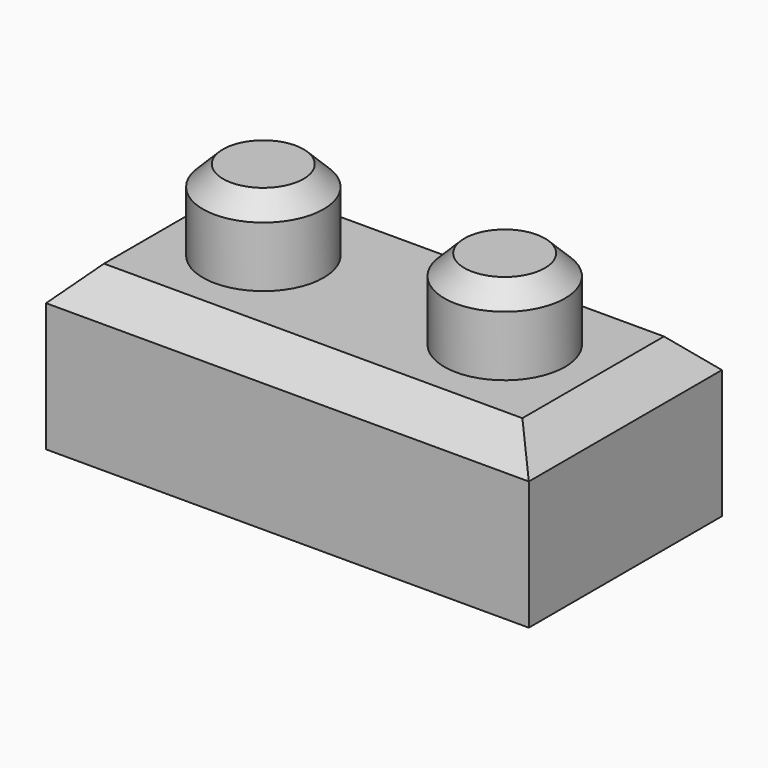
from build123d import *

# Parameters (mm, degrees)
F0_W     = 76.2
F0_H     = 38.1
F1_DEPTH = 25.4
F2_SIZE  = 5.08
F3_R     = 9.525
F4_DEPTH = 12.7
F5_SIZE2 = 3.175
F5_SIZE  = 3.175
F6_T     = 7.9375


# Not quite as in the source:
# - a shell that OpenCascade refuses in one call is made with other operations: the cavity is built on its own and cut out


with BuildPart() as f1:
    # F0 (on Top) → F1 (new body)
    with BuildSketch(Plane.XY):
        with Locations((38.1, -19.05)):
            Rectangle(F0_W, F0_H)
    extrude(amount=F1_DEPTH)

    # F2
    f2_edges = [f1.edges().sort_by_distance(p)[0] for p in [
        (38.1, -38.1, 25.4),
        (76.2, -19.05, 25.4),
        (38.1, 0, 25.4),
        (0, -19.05, 25.4),
    ]]
    chamfer(f2_edges, length=F2_SIZE)

    # F3 (on face) → F4 (join)
    with BuildSketch(Plane.XY.offset(25.4)):
        with Locations((19.05, -19.05)):
            Circle(F3_R)
        with Locations((57.15, -19.05)):
            Circle(F3_R)
    extrude(amount=F4_DEPTH)

    # F5
    f5_edges = [f1.edges().sort_by_distance(p)[0] for p in [
        (9.525, -19.05, 38.1),
        (47.625, -19.05, 38.1),
    ]]
    chamfer(f5_edges, length=F5_SIZE, length2=F5_SIZE2)

    # F6: shell of thickness 7.9375, made by hand


with BuildPart() as f6_core1:
    # F6_t2: copy of F1
    add(f1.part)

    # the walls: a layer under each face that stays
    f6_faces = [f6_core1.faces().sort_by_distance(p)[0] for p in [
        (9.525, -19.05, 30.1625),
        (11.1125, -19.05, 36.5125),
        (38.1, -19.05, 25.4),
        (19.05, -19.05, 38.1),
        (38.1, -35.56, 22.86),
        (2.54, -19.05, 22.86),
        (73.66, -19.05, 22.86),
        (38.1, -2.54, 22.86),
        (47.625, -19.05, 30.1625),
        (38.1, -38.1, 10.16),
        (0, -19.05, 10.16),
        (76.2, -19.05, 10.16),
        (38.1, 0, 10.16),
        (49.2125, -19.05, 36.5125),
        (57.15, -19.05, 38.1),
    ]]
    thicken(f6_faces, amount=-F6_T, mode=Mode.SUBTRACT)

    # F6_s3 → F6_t4 (revolve, cut)
    with BuildSketch(Plane.XZ.offset(19.05)):
        Polygon((28.654375, 25.479375), (20.6375, 25.4), (20.6375, 17.4625), (28.575, 17.4625), align=None)
    revolve(axis=Axis((19.05, -19.05, 25.4), (0, 0, 1)), mode=Mode.SUBTRACT)

    # F6_s5 → F6_t6 (revolve, cut)
    with BuildSketch(Plane.XZ.offset(19.05)):
        Polygon((66.754375, 25.479375), (66.675, 17.4625), (58.7375, 17.4625), (58.7375, 25.4), align=None)
    revolve(axis=Axis((57.15, -19.05, 25.4), (0, 0, 1)), mode=Mode.SUBTRACT)


with BuildPart() as f1_1:
    add(f1.part)

    # what is left inside the walls is the cavity
    f6_cavity = [f6_core1.part.solids().sort_by_distance(p)[0] for p in [
        (38.1, -22.754167, 0.079375),
    ]]
    add(f6_cavity, mode=Mode.SUBTRACT)


solid = f1_1.part
